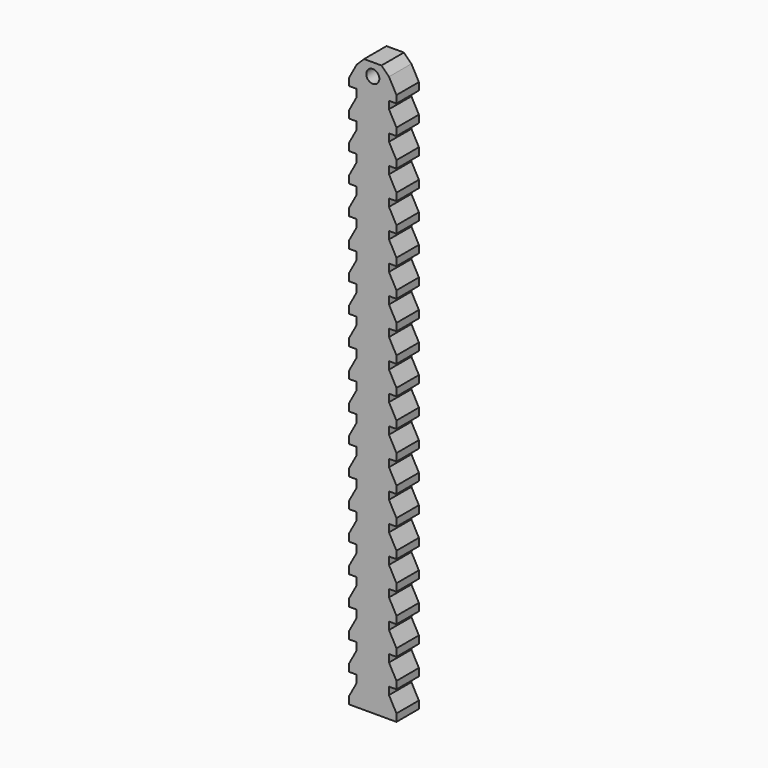
from build123d import *

# Parameters (mm, degrees)
F1_DEPTH = 4.5
F2_SIZE  = 1.19999
F3_R     = 1.05
F4_DEPTH = 25


# Not quite as in the source:
# - a fillet or chamfer is up to 0.001 mm smaller than in the source, because OpenCascade refuses the exact size


with BuildPart() as f1:
    # F0 (on Front) → F1 (new body)
    with BuildSketch(Plane.XZ):
        Polygon((-3.8, 1.2), (-3.8, 0), (-2.6, 0), (2.6, 0), (3.8, 0), (3.8, 1.2), (2.6, 3.4), (2.6, 4.6), (3.8, 4.6), (3.8, 5.8), (2.6, 8), (2.6, 9.2), (3.8, 9.2), (3.8, 10.4), (2.6, 12.6), (2.6, 13.8), (3.8, 13.8), (3.8, 15), (2.6, 17.2), (2.6, 18.4), (3.8, 18.4), (3.8, 19.6), (2.6, 21.8), (2.6, 23), (3.8, 23), (3.8, 24.2), (2.6, 26.4), (2.6, 27.6), (3.8, 27.6), (3.8, 28.8), (2.6, 31), (2.6, 32.2), (3.8, 32.2), (3.8, 33.4), (2.6, 35.6), (2.6, 36.8), (3.8, 36.8), (3.8, 38), (2.6, 40.2), (2.6, 41.4), (3.8, 41.4), (3.8, 42.6), (2.6, 44.8), (2.6, 46), (3.8, 46), (3.8, 47.2), (2.6, 49.4), (2.6, 50.6), (3.8, 50.6), (3.8, 51.8), (2.6, 54), (2.6, 55.2), (3.8, 55.2), (3.8, 56.4), (2.6, 58.6), (2.6, 59.8), (3.8, 59.8), (3.8, 61), (2.6, 63.2), (2.6, 64.4), (3.8, 64.4), (3.8, 65.6), (2.6, 67.8), (2.6, 69), (3.8, 69), (3.8, 70.2), (2.6, 72.4), (2.6, 73.6), (3.8, 73.6), (3.8, 74.8), (2.6, 77), (2.6, 78.2), (3.8, 78.2), (3.8, 79.4), (2.6, 81.6), (2.6, 82.8), (3.8, 82.8), (3.8, 84), (2.6, 86.2), (2.6, 87.4), (3.8, 87.4), (3.8, 88.6), (2.6, 90.8), (2.6, 92), (-2.6, 92), (-2.6, 90.8), (-3.8, 88.6), (-3.8, 87.4), (-2.6, 87.4), (-2.6, 86.2), (-3.8, 84), (-3.8, 82.8), (-2.6, 82.8), (-2.6, 81.6), (-3.8, 79.4), (-3.8, 78.2), (-2.6, 78.2), (-2.6, 77), (-3.8, 74.8), (-3.8, 73.6), (-2.6, 73.6), (-2.6, 72.4), (-3.8, 70.2), (-3.8, 69), (-2.6, 69), (-2.6, 67.8), (-3.8, 65.6), (-3.8, 64.4), (-2.6, 64.4), (-2.6, 63.2), (-3.8, 61), (-3.8, 59.8), (-2.6, 59.8), (-2.6, 58.6), (-3.8, 56.4), (-3.8, 55.2), (-2.6, 55.2), (-2.6, 54), (-3.8, 51.8), (-3.8, 50.6), (-2.6, 50.6), (-2.6, 49.4), (-3.8, 47.2), (-3.8, 46), (-2.6, 46), (-2.6, 44.8), (-3.8, 42.6), (-3.8, 41.4), (-2.6, 41.4), (-2.6, 40.2), (-3.8, 38), (-3.8, 36.8), (-2.6, 36.8), (-2.6, 35.6), (-3.8, 33.4), (-3.8, 32.2), (-2.6, 32.2), (-2.6, 31), (-3.8, 28.8), (-3.8, 27.6), (-2.6, 27.6), (-2.6, 26.4), (-3.8, 24.2), (-3.8, 23), (-2.6, 23), (-2.6, 21.8), (-3.8, 19.6), (-3.8, 18.4), (-2.6, 18.4), (-2.6, 17.2), (-3.8, 15), (-3.8, 13.8), (-2.6, 13.8), (-2.6, 12.6), (-3.8, 10.4), (-3.8, 9.2), (-2.6, 9.2), (-2.6, 8), (-3.8, 5.8), (-3.8, 4.6), (-2.6, 4.6), (-2.6, 3.4), align=None)
    extrude(amount=F1_DEPTH)

    # F2 (size 1.2 in the source; OpenCascade refuses exactly that, so slightly less here)
    f2_edges = [f1.edges().sort_by_distance(p)[0] for p in [
        (2.6, -2.25, 92),
        (-2.6, -2.25, 92),
    ]]
    chamfer(f2_edges, length=F2_SIZE)

    # F3 (on face) → F4 (cut)
    with BuildSketch(Plane.XZ.offset(4.5)):
        with Locations((0, 90)):
            Circle(F3_R)
    extrude(amount=-F4_DEPTH, mode=Mode.SUBTRACT)


solid = f1.part
